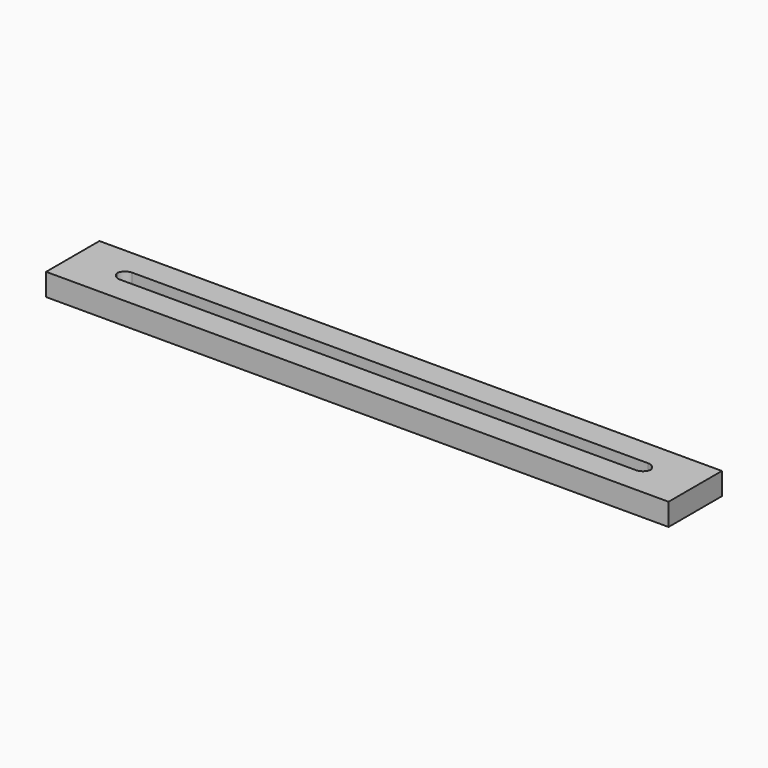
from build123d import *

# Parameters (mm, degrees)
F0_W        = 140
F0_H        = 15
F0_W_2      = 120
F0_H_2      = 3.4
F1_DEPTH    = 5
F2_T1_DEPTH = 5


# Not quite as in the source:
# - a fillet or chamfer that OpenCascade refuses, or shapes differently, is made with other operations: its cross-section is extruded or revolved along the edge and cut away or added


with BuildPart() as f1:
    # F0 (on Top) → F1 (new body)
    with BuildSketch(Plane.XY):
        Rectangle(F0_W, F0_H)
        Rectangle(F0_W_2, F0_H_2, mode=Mode.SUBTRACT)
    extrude(amount=F1_DEPTH)

    # F2: fillet of radius 2 on 4 edges, made by hand

    # F2_s2 → F2_t1 (join)
    with BuildSketch(Plane.XY):
        with BuildLine():
            ThreePointArc((-58, 1.7), (-59.4142135624, 1.1142135624), (-60, -0.3))
            Line((-60, -0.3), (-60, 1.7))
            Line((-60, 1.7), (-58, 1.7))
        make_face()
        with BuildLine():
            ThreePointArc((-58, -1.7), (-59.4142135624, -1.1142135624), (-60, 0.3))
            Line((-60, 0.3), (-60, -1.7))
            Line((-60, -1.7), (-58, -1.7))
        make_face()
        with BuildLine():
            ThreePointArc((58, 1.7), (59.4142135624, 1.1142135624), (60, -0.3))
            Line((60, -0.3), (60, 1.7))
            Line((60, 1.7), (58, 1.7))
        make_face()
        with BuildLine():
            ThreePointArc((60, 0.3), (59.4142135624, -1.1142135624), (58, -1.7))
            Line((58, -1.7), (60, -1.7))
            Line((60, -1.7), (60, 0.3))
        make_face()
    extrude(amount=F2_T1_DEPTH)


solid = f1.part
